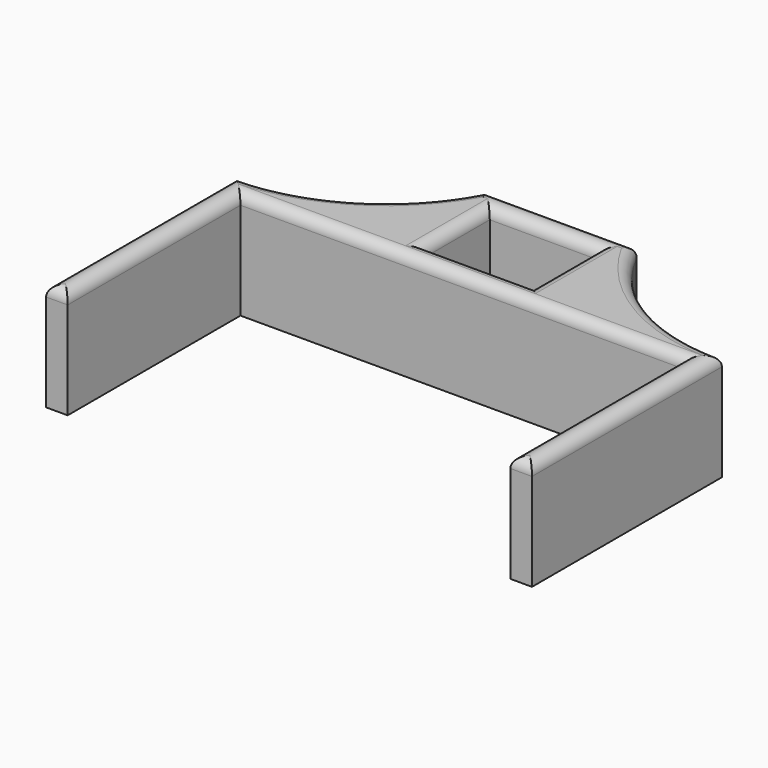
from build123d import *

# Parameters (mm, degrees)
F0_W         = 10
F0_H         = 7.5
F1_DEPTH     = 10
F2_T1_DEPTH  = 26.9846032165
F2_T3_DEPTH  = 7
F2_T5_DEPTH  = 22.5
F2_T7_DEPTH  = 41
F2_T9_DEPTH  = 7
F2_T11_DEPTH = 19
F2_T13_DEPTH = 7.5
F2_T15_DEPTH = 10
F2_T18_ANGLE = 79.4810617097
F2_T20_ANGLE = 79.4810617097
F2_T25_DEPTH = 25
F2_T29_DEPTH = 43.5
F2_T36_DEPTH = 43.5
F2_T40_DEPTH = 25
F2_T47_DEPTH = 10
F2_T51_DEPTH = 12.5
F2_T58_DEPTH = 10
F2_T62_DEPTH = 12.5
F2_T69_DEPTH = 12.5
F2_T73_DEPTH = 10
F2_T80_DEPTH = 10
F2_T84_DEPTH = 12.5


# Not quite as in the source:
# - a fillet or chamfer that OpenCascade refuses, or shapes differently, is made with other operations: its cross-section is extruded or revolved along the edge and cut away or added


with BuildPart() as f1:
    # F0 (on Top) → F1 (new body)
    with BuildSketch(Plane.XY):
        with BuildLine():
            Line((0, 34.8731837149), (41, 34.8731837149))
            Line((41, 34.8731837149), (41, 14.8731837149))
            Line((41, 14.8731837149), (43, 14.8731837149))
            Line((43, 14.8731837149), (43, 36.8577869315))
            ThreePointArc((43, 36.8577869315), (33.9101705187, 39.4217493566), (27.5, 46.3577869315))
            Line((27.5, 46.3577869315), (13.5, 46.3577869315))
            ThreePointArc((13.5, 46.3577869315), (7.0898294813, 39.4217493566), (-2, 36.8577869315))
            Line((-2, 36.8577869315), (-2, 14.8731837149))
            Line((-2, 14.8731837149), (0, 14.8731837149))
            Line((0, 14.8731837149), (0, 34.8731837149))
        make_face()
        with Locations((20.5, 40.6077869315)):
            Rectangle(F0_W, F0_H, mode=Mode.SUBTRACT)
    extrude(amount=F1_DEPTH)

    # F2: fillet of radius 1 on 14 edges, made by hand

    # F2_s2 → F2_t1 (cut)
    with BuildSketch(Plane.XZ.offset(-39.3577869315)):
        with BuildLine():
            ThreePointArc((-2, 9), (-1.7071067812, 9.7071067812), (-1, 10))
            Line((-1, 10), (-2, 10))
            Line((-2, 10), (-2, 9))
        make_face()
        with BuildLine():
            ThreePointArc((43, 9), (42.7071067812, 9.7071067812), (42, 10))
            Line((42, 10), (43, 10))
            Line((43, 10), (43, 9))
        make_face()
    extrude(amount=F2_T1_DEPTH, mode=Mode.SUBTRACT)

    # F2_s4 → F2_t3 (cut)
    with BuildSketch(Plane.YZ.offset(-4.5)):
        with BuildLine():
            ThreePointArc((14.8731837149, 9), (15.1660769337, 9.7071067812), (15.8731837149, 10))
            Line((15.8731837149, 10), (14.8731837149, 10))
            Line((14.8731837149, 10), (14.8731837149, 9))
        make_face()
    extrude(amount=F2_T3_DEPTH, mode=Mode.SUBTRACT)

    # F2_s6 → F2_t5 (cut)
    with BuildSketch(Plane.XZ.offset(-34.8731837149)):
        with BuildLine():
            ThreePointArc((0, 9), (-0.2928932188, 9.7071067812), (-1, 10))
            Line((-1, 10), (0, 10))
            Line((0, 10), (0, 9))
        make_face()
        with BuildLine():
            ThreePointArc((41, 9), (41.2928932188, 9.7071067812), (42, 10))
            Line((42, 10), (41, 10))
            Line((41, 10), (41, 9))
        make_face()
    extrude(amount=F2_T5_DEPTH, mode=Mode.SUBTRACT)

    # F2_s8 → F2_t7 (cut)
    with BuildSketch(Plane.YZ):
        with BuildLine():
            ThreePointArc((34.8731837149, 9), (35.1660769337, 9.7071067812), (35.8731837149, 10))
            Line((35.8731837149, 10), (34.8731837149, 10))
            Line((34.8731837149, 10), (34.8731837149, 9))
        make_face()
    extrude(amount=F2_T7_DEPTH, mode=Mode.SUBTRACT)

    # F2_s10 → F2_t9 (cut)
    with BuildSketch(Plane.YZ.offset(38.5)):
        with BuildLine():
            ThreePointArc((14.8731837149, 9), (15.1660769337, 9.7071067812), (15.8731837149, 10))
            Line((15.8731837149, 10), (14.8731837149, 10))
            Line((14.8731837149, 10), (14.8731837149, 9))
        make_face()
    extrude(amount=F2_T9_DEPTH, mode=Mode.SUBTRACT)

    # F2_s12 → F2_t11 (cut)
    with BuildSketch(Plane.YZ.offset(11)):
        with BuildLine():
            ThreePointArc((46.3577869315, 9), (46.0648937127, 9.7071067812), (45.3577869315, 10))
            Line((45.3577869315, 10), (46.3577869315, 10))
            Line((46.3577869315, 10), (46.3577869315, 9))
        make_face()
    extrude(amount=F2_T11_DEPTH, mode=Mode.SUBTRACT)

    # F2_s14 → F2_t13 (cut)
    with BuildSketch(Plane.XZ.offset(-44.3577869315)):
        with BuildLine():
            ThreePointArc((25.5, 9), (25.7928932188, 9.7071067812), (26.5, 10))
            Line((26.5, 10), (25.5, 10))
            Line((25.5, 10), (25.5, 9))
        make_face()
        with BuildLine():
            ThreePointArc((15.5, 9), (15.2071067812, 9.7071067812), (14.5, 10))
            Line((14.5, 10), (15.5, 10))
            Line((15.5, 10), (15.5, 9))
        make_face()
    extrude(amount=F2_T13_DEPTH, mode=Mode.SUBTRACT)

    # F2_s16 → F2_t15 (cut)
    with BuildSketch(Plane.YZ.offset(15.5)):
        with BuildLine():
            ThreePointArc((36.8577869315, 9), (36.5648937127, 9.7071067812), (35.8577869315, 10))
            Line((35.8577869315, 10), (36.8577869315, 10))
            Line((36.8577869315, 10), (36.8577869315, 9))
        make_face()
        with BuildLine():
            ThreePointArc((44.3577869315, 9), (44.6506801503, 9.7071067812), (45.3577869315, 10))
            Line((45.3577869315, 10), (44.3577869315, 10))
            Line((44.3577869315, 10), (44.3577869315, 9))
        make_face()
    extrude(amount=F2_T15_DEPTH, mode=Mode.SUBTRACT)

    # F2_s17 → F2_t18 (revolve, cut)
    with BuildSketch(Plane(origin=(16.3105725922, 48.0350676987, 0), x_dir=(0, 0, 1), z_dir=(0.3215254447, 0.9469009391, 0))):
        with BuildLine():
            ThreePointArc((9, -1.9426318697), (9.7071067812, -1.6497386509), (10, -0.9426318697))
            Line((10, -0.9426318697), (10, -1.9426318697))
            Line((10, -1.9426318697), (9, -1.9426318697))
        make_face()
    revolve(axis=Axis((-2, 54.2525237736, 10), (0, 0, -1)), revolution_arc=F2_T18_ANGLE, mode=Mode.SUBTRACT)

    # F2_s19 → F2_t20 (revolve, cut)
    with BuildSketch(Plane(origin=(49.8093527962, 7.2098207335, 0), x_dir=(0, 0, 1), z_dir=(0.9896857587, 0.1432553627, 0))):
        with BuildLine():
            ThreePointArc((9, -30.138232714), (9.7071067812, -29.8453394951), (10, -29.138232714))
            Line((10, -29.138232714), (10, -30.138232714))
            Line((10, -30.138232714), (9, -30.138232714))
        make_face()
    revolve(axis=Axis((43, 54.2525237736, 10), (0, 0, -1)), revolution_arc=F2_T20_ANGLE, mode=Mode.SUBTRACT)


with BuildPart() as f2_tool23:
    # F2_s24 → F2_t25 (new body)
    with BuildSketch(Plane.XZ.offset(-12.3731837149)):
        with BuildLine():
            ThreePointArc((0, 9), (-0.2928932188, 9.7071067812), (-1, 10))
            Line((-1, 10), (0, 10))
            Line((0, 10), (0, 9))
        make_face()
    extrude(amount=-F2_T25_DEPTH)

    split(bisect_by=Plane.XZ.offset(-34.8731837149), keep=Keep.BOTTOM)


with BuildPart() as f2_tool27:
    # F2_s28 → F2_t29 (new body)
    with BuildSketch(Plane.YZ.offset(-2.5)):
        with BuildLine():
            ThreePointArc((34.8731837149, 9), (35.1660769337, 9.7071067812), (35.8731837149, 10))
            Line((35.8731837149, 10), (34.8731837149, 10))
            Line((34.8731837149, 10), (34.8731837149, 9))
        make_face()
    extrude(amount=F2_T29_DEPTH)

    split(bisect_by=Plane.YZ, keep=Keep.BOTTOM)


with BuildPart() as f2_tool23_1:
    add(f2_tool23.part)

    # F2_t31: intersect F2_tool27
    add(f2_tool27.part, mode=Mode.INTERSECT)


with BuildPart() as f1_1:
    add(f1.part)

    # F2_t21: cut F2_tool23
    add(f2_tool23_1.part, mode=Mode.SUBTRACT)


with BuildPart() as f2_tool34:
    # F2_s35 → F2_t36 (new body)
    with BuildSketch(Plane.YZ):
        with BuildLine():
            ThreePointArc((34.8731837149, 9), (35.1660769337, 9.7071067812), (35.8731837149, 10))
            Line((35.8731837149, 10), (34.8731837149, 10))
            Line((34.8731837149, 10), (34.8731837149, 9))
        make_face()
    extrude(amount=F2_T36_DEPTH)

    split(bisect_by=Plane.YZ.offset(41), keep=Keep.TOP)


with BuildPart() as f2_tool38:
    # F2_s39 → F2_t40 (new body)
    with BuildSketch(Plane.XZ.offset(-37.3731837149)):
        with BuildLine():
            ThreePointArc((41, 9), (41.2928932188, 9.7071067812), (42, 10))
            Line((42, 10), (41, 10))
            Line((41, 10), (41, 9))
        make_face()
    extrude(amount=F2_T40_DEPTH)

    split(bisect_by=Plane.XZ.offset(-34.8731837149), keep=Keep.BOTTOM)


with BuildPart() as f2_tool34_1:
    add(f2_tool34.part)

    # F2_t42: intersect F2_tool38
    add(f2_tool38.part, mode=Mode.INTERSECT)


with BuildPart() as f1_2:
    add(f1_1.part)

    # F2_t32: cut F2_tool34
    add(f2_tool34_1.part, mode=Mode.SUBTRACT)


with BuildPart() as f2_tool45:
    # F2_s46 → F2_t47 (new body)
    with BuildSketch(Plane.XZ.offset(-46.8577869315)):
        with BuildLine():
            ThreePointArc((25.5, 9), (25.7928932188, 9.7071067812), (26.5, 10))
            Line((26.5, 10), (25.5, 10))
            Line((25.5, 10), (25.5, 9))
        make_face()
    extrude(amount=F2_T47_DEPTH)

    split(bisect_by=Plane.XZ.offset(-44.3577869315), keep=Keep.BOTTOM)


with BuildPart() as f2_tool49:
    # F2_s50 → F2_t51 (new body)
    with BuildSketch(Plane.YZ.offset(15.5)):
        with BuildLine():
            ThreePointArc((44.3577869315, 9), (44.6506801503, 9.7071067812), (45.3577869315, 10))
            Line((45.3577869315, 10), (44.3577869315, 10))
            Line((44.3577869315, 10), (44.3577869315, 9))
        make_face()
    extrude(amount=F2_T51_DEPTH)

    split(bisect_by=Plane.YZ.offset(25.5), keep=Keep.TOP)


with BuildPart() as f2_tool45_1:
    add(f2_tool45.part)

    # F2_t53: intersect F2_tool49
    add(f2_tool49.part, mode=Mode.INTERSECT)


with BuildPart() as f1_3:
    add(f1_2.part)

    # F2_t43: cut F2_tool45
    add(f2_tool45_1.part, mode=Mode.SUBTRACT)


with BuildPart() as f2_tool56:
    # F2_s57 → F2_t58 (new body)
    with BuildSketch(Plane.XZ.offset(-44.3577869315)):
        with BuildLine():
            ThreePointArc((25.5, 9), (25.7928932188, 9.7071067812), (26.5, 10))
            Line((26.5, 10), (25.5, 10))
            Line((25.5, 10), (25.5, 9))
        make_face()
    extrude(amount=F2_T58_DEPTH)

    split(bisect_by=Plane.XZ.offset(-36.8577869315), keep=Keep.TOP)


with BuildPart() as f2_tool60:
    # F2_s61 → F2_t62 (new body)
    with BuildSketch(Plane.YZ.offset(28)):
        with BuildLine():
            ThreePointArc((36.8577869315, 9), (36.5648937127, 9.7071067812), (35.8577869315, 10))
            Line((35.8577869315, 10), (36.8577869315, 10))
            Line((36.8577869315, 10), (36.8577869315, 9))
        make_face()
    extrude(amount=-F2_T62_DEPTH)

    split(bisect_by=Plane.YZ.offset(25.5), keep=Keep.TOP)


with BuildPart() as f2_tool56_1:
    add(f2_tool56.part)

    # F2_t64: intersect F2_tool60
    add(f2_tool60.part, mode=Mode.INTERSECT)


with BuildPart() as f1_4:
    add(f1_3.part)

    # F2_t54: cut F2_tool56
    add(f2_tool56_1.part, mode=Mode.SUBTRACT)


with BuildPart() as f2_tool67:
    # F2_s68 → F2_t69 (new body)
    with BuildSketch(Plane.YZ.offset(25.5)):
        with BuildLine():
            ThreePointArc((36.8577869315, 9), (36.5648937127, 9.7071067812), (35.8577869315, 10))
            Line((35.8577869315, 10), (36.8577869315, 10))
            Line((36.8577869315, 10), (36.8577869315, 9))
        make_face()
    extrude(amount=-F2_T69_DEPTH)

    split(bisect_by=Plane.YZ.offset(15.5), keep=Keep.BOTTOM)


with BuildPart() as f2_tool71:
    # F2_s72 → F2_t73 (new body)
    with BuildSketch(Plane.XZ.offset(-34.3577869315)):
        with BuildLine():
            ThreePointArc((15.5, 9), (15.2071067812, 9.7071067812), (14.5, 10))
            Line((14.5, 10), (15.5, 10))
            Line((15.5, 10), (15.5, 9))
        make_face()
    extrude(amount=-F2_T73_DEPTH)

    split(bisect_by=Plane.XZ.offset(-36.8577869315), keep=Keep.TOP)


with BuildPart() as f2_tool67_1:
    add(f2_tool67.part)

    # F2_t75: intersect F2_tool71
    add(f2_tool71.part, mode=Mode.INTERSECT)


with BuildPart() as f1_5:
    add(f1_4.part)

    # F2_t65: cut F2_tool67
    add(f2_tool67_1.part, mode=Mode.SUBTRACT)


with BuildPart() as f2_tool78:
    # F2_s79 → F2_t80 (new body)
    with BuildSketch(Plane.XZ.offset(-36.8577869315)):
        with BuildLine():
            ThreePointArc((15.5, 9), (15.2071067812, 9.7071067812), (14.5, 10))
            Line((14.5, 10), (15.5, 10))
            Line((15.5, 10), (15.5, 9))
        make_face()
    extrude(amount=-F2_T80_DEPTH)

    split(bisect_by=Plane.XZ.offset(-44.3577869315), keep=Keep.BOTTOM)


with BuildPart() as f2_tool82:
    # F2_s83 → F2_t84 (new body)
    with BuildSketch(Plane.YZ.offset(13)):
        with BuildLine():
            ThreePointArc((44.3577869315, 9), (44.6506801503, 9.7071067812), (45.3577869315, 10))
            Line((45.3577869315, 10), (44.3577869315, 10))
            Line((44.3577869315, 10), (44.3577869315, 9))
        make_face()
    extrude(amount=F2_T84_DEPTH)

    split(bisect_by=Plane.YZ.offset(15.5), keep=Keep.BOTTOM)


with BuildPart() as f2_tool78_1:
    add(f2_tool78.part)

    # F2_t86: intersect F2_tool82
    add(f2_tool82.part, mode=Mode.INTERSECT)


with BuildPart() as f1_6:
    add(f1_5.part)

    # F2_t76: cut F2_tool78
    add(f2_tool78_1.part, mode=Mode.SUBTRACT)


solid = f1_6.part
